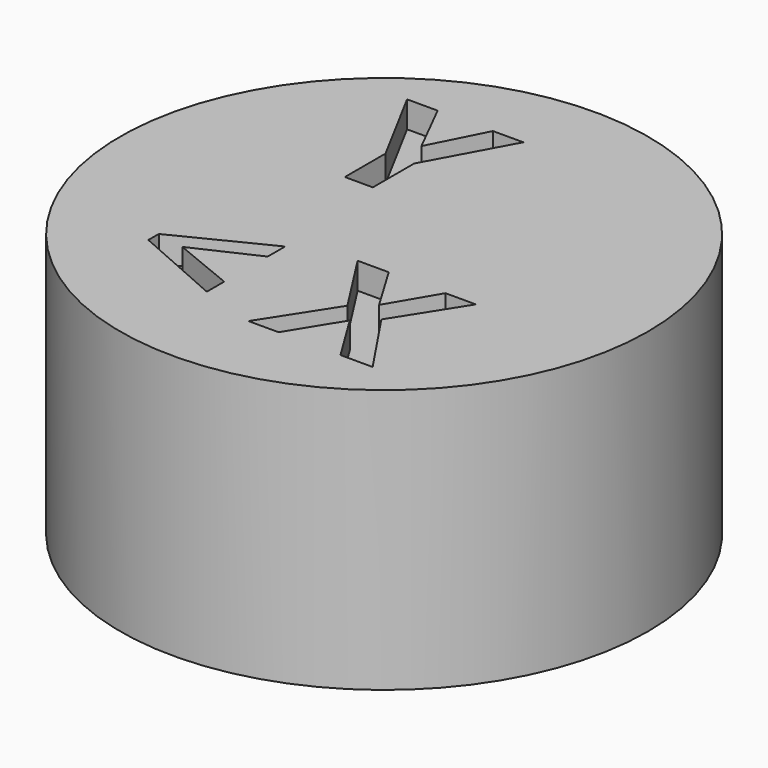
from build123d import *

# Parameters (mm, degrees)
F0_R         = 10
F1_DEPTH     = 10
F2_TEXT_SIZE = 7.0555555556
F3_DEPTH     = 1


# Not quite as in the source:
# - Text() gives the source's letters only with a copy of the font that has no kerning and outlines rounded to 1/6400 em; it was checked with that copy


with BuildPart() as f1:
    # F0 (on Top) → F1 (new body)
    with BuildSketch(Plane.XY):
        Circle(F0_R)
    extrude(amount=F1_DEPTH)

    # F2 (on face) → F3 (cut)
    with BuildSketch(Plane.XY.offset(10)):
        with Locations((-5.5121527778, -6.8609635628)):
            Text('< X', F2_TEXT_SIZE, font='Open Sans', font_style=FontStyle.BOLD, text_align=(TextAlign.LEFT, TextAlign.BOTTOM))
        with Locations((-4.8606163194, 2.1265231098)):
            Text('Y', F2_TEXT_SIZE, font='Open Sans', font_style=FontStyle.BOLD, text_align=(TextAlign.LEFT, TextAlign.BOTTOM))
    extrude(amount=-F3_DEPTH, mode=Mode.SUBTRACT)


solid = f1.part
